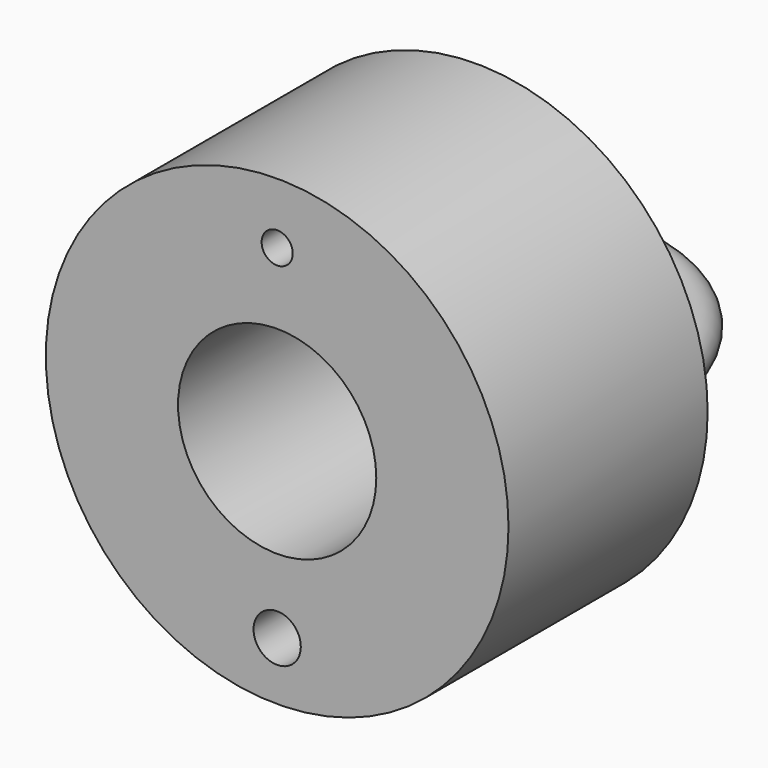
from build123d import *

# Parameters (mm, degrees)
F0_R     = 47.2126506678
F0_R_2   = 20.2272154061
F1_DEPTH = 50.8
F2_R     = 3.175
F2_R_2   = 4.8238037601
F3_DEPTH = 50.801
F4_R     = 4.3834323194
F5_ANGLE = 180


# Not quite as in the source:
# - the program builds the solid bodies; features that only make, move or delete a surface that nothing else refers to are left out


with BuildPart() as f1:
    # F0 (on Front) → F1 (new body)
    with BuildSketch(Plane.XZ):
        Circle(F0_R)
        Circle(F0_R_2, mode=Mode.SUBTRACT)
    extrude(amount=F1_DEPTH)

    # F2 (on Front) → F3 (cut, through all)
    with BuildSketch(Plane.XZ):
        with Locations((0, 34.7616262734)):
            Circle(F2_R)
        with Locations((0, -35.3442244232)):
            Circle(F2_R_2)
    extrude(amount=F3_DEPTH, mode=Mode.SUBTRACT)

    # F4 (on Front) → F5 (revolve)
    with BuildSketch(Plane.XZ):
        with Locations((-34.811783582, 0)):
            Circle(F4_R)
    revolve(axis=Axis((0, 0, 1.5608235262), (0, 0, -1)), revolution_arc=F5_ANGLE)


solid = f1.part
